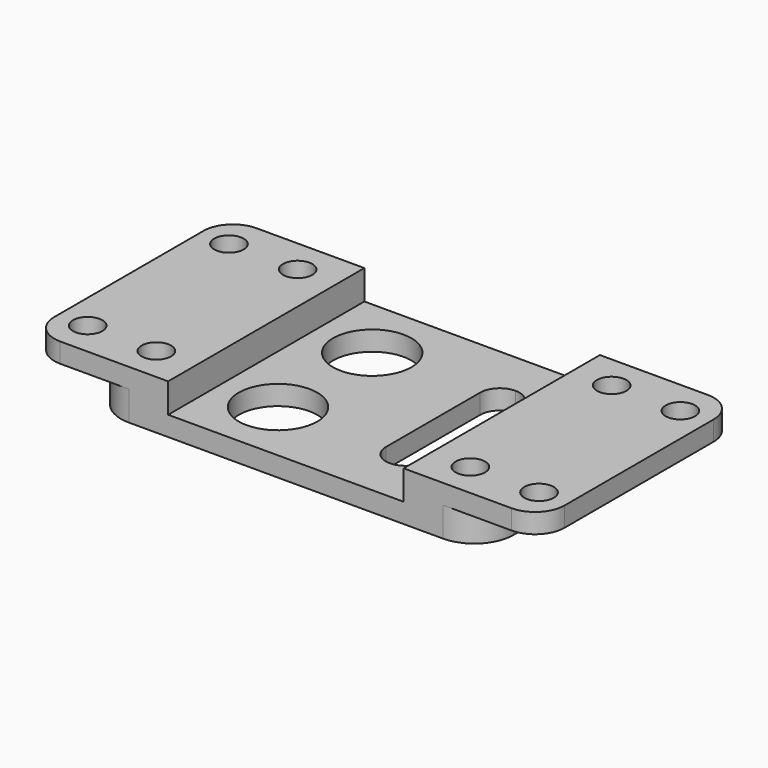
from build123d import *

# Parameters (mm, degrees)
F0_W      = 40
F0_H      = 25
F1_DEPTH  = 3
F2_R      = 4
F3_W      = 52
F3_H      = 25
F4_DEPTH  = 2
F5_R      = 3
F6_R      = 1.5
F7_DEPTH  = 25
F8_R      = 1.5
F9_DEPTH  = 4
F10_W     = 24
F10_H     = 25
F11_DEPTH = 3
F12_W     = 4
F12_H     = 16
F12_R     = 4
F13_DEPTH = 25
F14_R     = 1.99999


# Not quite as in the source:
# - a fillet or chamfer is up to 0.001 mm smaller than in the source, because OpenCascade refuses the exact size


with BuildPart() as f1:
    # F0 (on Top) → F1 (new body)
    with BuildSketch(Plane.XY):
        Rectangle(F0_W, F0_H)
    extrude(amount=F1_DEPTH)

    # F2
    f2_edges = [f1.edges().sort_by_distance(p)[0] for p in [
        (-20, -12.5, 1.5),
        (-20, 12.5, 1.5),
        (20, -12.5, 1.5),
        (20, 12.5, 1.5),
    ]]
    fillet(f2_edges, radius=F2_R)

    # F3 (on face) → F4 (join)
    with BuildSketch(Plane.XY.offset(3)):
        Rectangle(F3_W, F3_H)
    extrude(amount=F4_DEPTH)

    # F5
    f5_edges = [f1.edges().sort_by_distance(p)[0] for p in [
        (26, 12.5, 4),
        (26, -12.5, 4),
        (-26, -12.5, 4),
        (-26, 12.5, 4),
    ]]
    fillet(f5_edges, radius=F5_R)

    # F6 (on Top) → F7 (cut)
    with BuildSketch(Plane.XY):
        with Locations((23, 9)):
            Circle(F6_R)
        with Locations((23, -9)):
            Circle(F6_R)
        with Locations((-23, -9)):
            Circle(F6_R)
        with Locations((-23, 9)):
            Circle(F6_R)
    extrude(amount=F7_DEPTH, mode=Mode.SUBTRACT)

    # F8 (on face) → F9 (cut)
    with BuildSketch(Plane.XY.offset(5)):
        with Locations((16, -9)):
            Circle(F8_R)
        with Locations((-16, -9)):
            Circle(F8_R)
        with Locations((-16, 9)):
            Circle(F8_R)
        with Locations((16, 9)):
            Circle(F8_R)
    extrude(amount=-F9_DEPTH, mode=Mode.SUBTRACT)

    # F10 (on face) → F11 (cut)
    with BuildSketch(Plane.XY.offset(5)):
        Rectangle(F10_W, F10_H)
    extrude(amount=-F11_DEPTH, mode=Mode.SUBTRACT)

    # F12 (on face) → F13 (cut)
    with BuildSketch(Plane(origin=(0, 0, 0), x_dir=(1, 0, 0), z_dir=(0, 0, -1))):
        with Locations((7, 0)):
            Rectangle(F12_W, F12_H)
        with Locations((-6, -6)):
            Circle(F12_R)
        with Locations((-6, 6)):
            Circle(F12_R)
    extrude(amount=-F13_DEPTH, mode=Mode.SUBTRACT)

    # F14 (radius 2 in the source; OpenCascade refuses exactly that, so slightly less here)
    f14_edges = [f1.edges().sort_by_distance(p)[0] for p in [
        (9, 8, 1),
        (5, 8, 1),
        (9, -8, 1),
        (5, -8, 1),
    ]]
    fillet(f14_edges, radius=F14_R)


solid = f1.part
